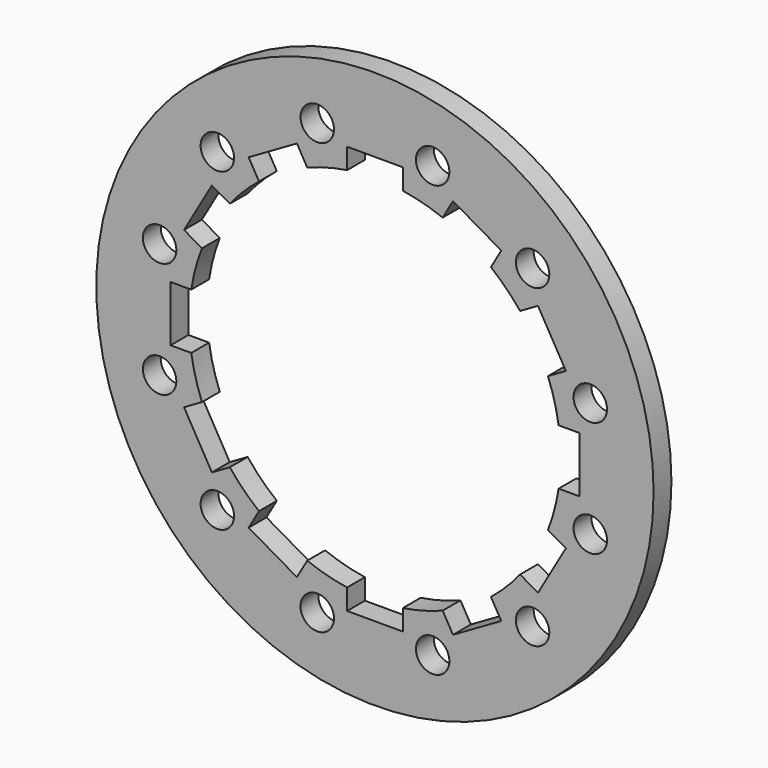
from build123d import *

# Parameters (mm, degrees)
F1_R            = 75
F1_R_2          = 50
F2_DEPTH        = 3
F4_DEPTH        = 35
F4_COPIES_COUNT = 12
F5_R            = 4.5
F6_DEPTH        = 12.5
F6_COPIES_COUNT = 12


# Not quite as in the source:
# - a pattern or mirror of a feature is missing from the dataset's text; its kind, count and spacing are read off the source's solid


with BuildPart() as f2:
    # F1 (on Front) → F2 (new body, symmetric)
    with BuildSketch(Plane.XZ):
        Circle(F1_R)
        Circle(F1_R_2, mode=Mode.SUBTRACT)
    extrude(amount=F2_DEPTH, both=True)

    # F3 (on face) → F4 (cut)
    with BuildSketch(Plane.XZ.offset(3)):
        with BuildLine():
            Line((-7.5, 49.4342998332), (-7.5, 0))
            Line((-7.5, 0), (7.5, 0))
            Line((7.5, 0), (7.5, 49.4342998332))
            ThreePointArc((7.5, 49.4342998332), (0, 50), (-7.5, 49.4342998332))
        make_face()
        with BuildLine():
            Line((-7.5, 55), (-7.5, 49.4342998332))
            ThreePointArc((-7.5, 49.4342998332), (0, 50), (7.5, 49.4342998332))
            Line((7.5, 49.4342998332), (7.5, 55))
            Line((7.5, 55), (-7.5, 55))
        make_face()
    f4 = extrude(amount=-F4_DEPTH, mode=Mode.SUBTRACT)

    # F4_copies: F4 ×12 about axis
    f4_copies_axis = Axis((0, 0, 0), (0, 1, 0))
    for i in range(1, F4_COPIES_COUNT):
        add(f4.rotate(f4_copies_axis, i * 360 / F4_COPIES_COUNT), mode=Mode.SUBTRACT)

    # F5 (on Front) → F6 (cut, symmetric)
    with BuildSketch(Plane.XZ):
        with Locations((42.4264068712, 42.4264068712)):
            Circle(F5_R)
    f6 = extrude(amount=F6_DEPTH, both=True, mode=Mode.SUBTRACT)

    # F6_copies: F6 ×12 about axis
    f6_copies_axis = Axis((0, 0, 0), (0, 1, 0))
    for i in range(1, F6_COPIES_COUNT):
        add(f6.rotate(f6_copies_axis, i * 360 / F6_COPIES_COUNT), mode=Mode.SUBTRACT)


solid = f2.part
